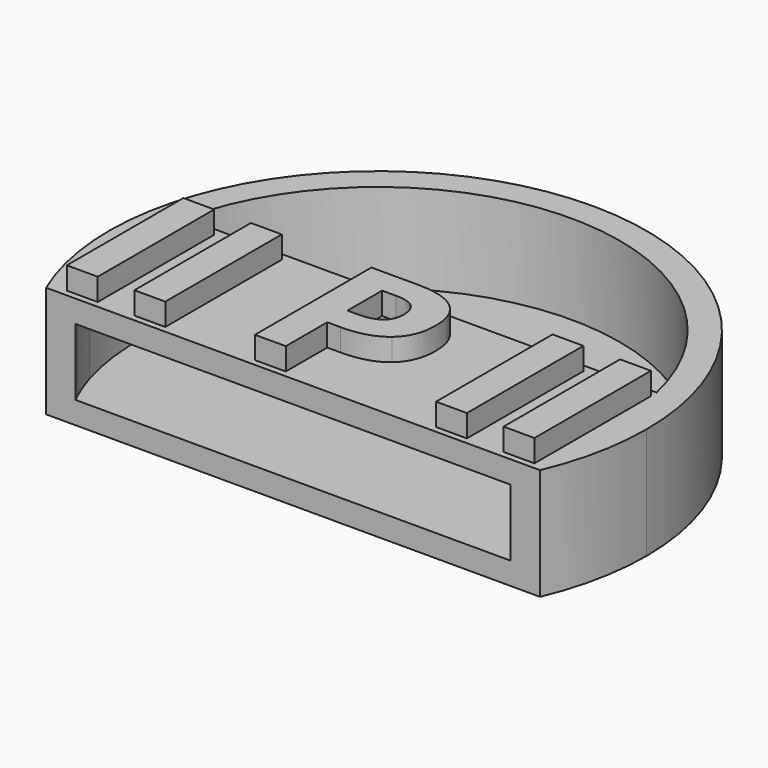
from build123d import *

# Parameters (mm, degrees)
F0_W     = 1.3848739799
F0_H     = 6.5299166297
F1_DEPTH = 5
F2_DEPTH = 6
F3_DEPTH = 4
F4_DEPTH = 1


# Not quite as in the source:
# - a feature names something its author has since deleted; it is built from what else it names


with BuildPart() as f1:
    # F0 (on Top) → F1 (new body)
    with BuildSketch(Plane.XY):
        with BuildLine():
            ThreePointArc((-9.8874952566, -4.4676545918), (-9.8222615585, -4.6093034047), (-9.7549987186, -4.75))
            Line((-9.7549987186, -4.75), (9.7549987186, -4.75))
            ThreePointArc((9.7549987186, -4.75), (9.8222615585, -4.6093034047), (9.8874952566, -4.4676545918))
            Line((9.8874952566, -4.4676545918), (9.2131992894, -4.4676545918))
            Line((9.2131992894, -4.4676545918), (9.2131992894, 2.062262038))
            Line((9.2131992894, 2.062262038), (10.5980732693, 2.062262038))
            Line((10.5980732693, 2.062262038), (10.5980732693, -2.3245091907))
            ThreePointArc((10.5980732693, -2.3245091907), (10.7868344516, -1.1690605262), (10.85, 0))
            ThreePointArc((10.85, 0), (10.7825989969, 1.2075010861), (10.5812333875, 2.4))
            Line((10.5812333875, 2.4), (0, 2.4))
            Line((0, 2.4), (-10.5812333875, 2.4))
            ThreePointArc((-10.5812333875, 2.4), (-10.8422277422, -0.4106063639), (-10.3694047071, -3.1934223053))
            Line((-10.3694047071, -3.1934223053), (-10.3694047071, 2.062262038))
            Line((-10.3694047071, 2.062262038), (-8.9845307272, 2.062262038))
            Line((-8.9845307272, 2.062262038), (-8.9845307272, -4.4676545918))
            Line((-8.9845307272, -4.4676545918), (-9.8874952566, -4.4676545918))
        make_face()
        with Locations((-6.6485384464, -1.2026962769)):
            Rectangle(F0_W, F0_H, mode=Mode.SUBTRACT)
        with BuildLine():
            add(Edge.make_bspline(
                [(1.9565453854, 1.55061613), (2.5746650927, 1.0389702221), (2.5746650927, 0.0256826557)],
                knots=[0, 0, 0, 1, 1, 1], degree=2))
            add(Edge.make_bspline(
                [(2.5746650927, 0.0256826557), (2.5746650927, -1.0290510875), (1.9158137978, -1.5871452971)],
                knots=[0, 0, 0, 1, 1, 1], degree=2))
            add(Edge.make_bspline(
                [(1.9158137978, -1.5871452971), (1.2569625029, -2.1452395068), (0.0421607662, -2.1452395068)],
                knots=[0, 0, 0, 1, 1, 1], degree=2))
            Line((0.0421607662, -2.1452395068), (-0.5509483171, -2.1452395068))
            Line((-0.5509483171, -2.1452395068), (-0.5509483171, -4.4676545918))
            Line((-0.5509483171, -4.4676545918), (-1.935822297, -4.4676545918))
            Line((-1.935822297, -4.4676545918), (-1.935822297, 2.062262038))
            Line((-1.935822297, 2.062262038), (0.1493491547, 2.062262038))
            add(Edge.make_bspline(
                [(0.1493491547, 2.062262038), (1.3384256782, 2.062262038), (1.9565453854, 1.55061613)],
                knots=[0, 0, 0, 1, 1, 1], degree=2))
        make_face(mode=Mode.SUBTRACT)
        with Locations((6.8772070086, -1.2026962769)):
            Rectangle(F0_W, F0_H, mode=Mode.SUBTRACT)
        with BuildLine():
            ThreePointArc((11.0742945599, -4.75), (11.8035534787, -2.4245876508), (12.05, 0))
            ThreePointArc((12.05, 0), (-2.4245876508, 11.8035534787), (-11.0742945599, -4.75))
            Line((-11.0742945599, -4.75), (-9.7549987186, -4.75))
            ThreePointArc((-9.7549987186, -4.75), (-9.8222615585, -4.6093034047), (-9.8874952566, -4.4676545918))
            Line((-9.8874952566, -4.4676545918), (-10.3694047071, -4.4676545918))
            Line((-10.3694047071, -4.4676545918), (-10.3694047071, -3.1934223053))
            ThreePointArc((-10.3694047071, -3.1934223053), (-10.8422277422, -0.4106063639), (-10.5812333875, 2.4))
            ThreePointArc((-10.5812333875, 2.4), (0, 10.85), (10.5812333875, 2.4))
            ThreePointArc((10.5812333875, 2.4), (10.7825989969, 1.2075010861), (10.85, 0))
            ThreePointArc((10.85, 0), (10.7868344516, -1.1690605262), (10.5980732693, -2.3245091907))
            Line((10.5980732693, -2.3245091907), (10.5980732693, -4.4676545918))
            Line((10.5980732693, -4.4676545918), (9.8874952566, -4.4676545918))
            ThreePointArc((9.8874952566, -4.4676545918), (9.8222615585, -4.6093034047), (9.7549987186, -4.75))
            Line((9.7549987186, -4.75), (11.0742945599, -4.75))
        make_face()
        with BuildLine():
            Line((-0.5509483171, 0.927494298), (-0.5509483171, -1.0104717668))
            Line((-0.5509483171, -1.0104717668), (-0.0950403712, -1.0104717668))
            add(Edge.make_bspline(
                [(-0.0950403712, -1.0104717668), (0.542373246, -1.0104717668), (0.8596508761, -0.7582217591)],
                knots=[0, 0, 0, 1, 1, 1], degree=2))
            add(Edge.make_bspline(
                [(0.8596508761, -0.7582217591), (1.1769285061, -0.5059717514), (1.1769285061, -0.0243385922)],
                knots=[0, 0, 0, 1, 1, 1], degree=2))
            add(Edge.make_bspline(
                [(1.1769285061, -0.0243385922), (1.1769285061, 0.463011281), (0.9111013026, 0.6952527895)],
                knots=[0, 0, 0, 1, 1, 1], degree=2))
            add(Edge.make_bspline(
                [(0.9111013026, 0.6952527895), (0.645274099, 0.927494298), (0.077890229, 0.927494298)],
                knots=[0, 0, 0, 1, 1, 1], degree=2))
            Line((0.077890229, 0.927494298), (-0.5509483171, 0.927494298))
        make_face()
    extrude(amount=F1_DEPTH)

    # F0 (on Top) → F2 (join)
    with BuildSketch(Plane.XY):
        with BuildLine():
            ThreePointArc((-10.3694047071, -3.1934223053), (-10.1484686537, -3.8381094285), (-9.8874952566, -4.4676545918))
            Line((-9.8874952566, -4.4676545918), (-8.9845307272, -4.4676545918))
            Line((-8.9845307272, -4.4676545918), (-8.9845307272, 2.062262038))
            Line((-8.9845307272, 2.062262038), (-10.3694047071, 2.062262038))
            Line((-10.3694047071, 2.062262038), (-10.3694047071, -3.1934223053))
        make_face()
        with BuildLine():
            Line((-10.3694047071, -4.4676545918), (-9.8874952566, -4.4676545918))
            ThreePointArc((-9.8874952566, -4.4676545918), (-10.1484686537, -3.8381094285), (-10.3694047071, -3.1934223053))
            Line((-10.3694047071, -3.1934223053), (-10.3694047071, -4.4676545918))
        make_face()
        with Locations((-6.6485384464, -1.2026962769)):
            Rectangle(F0_W, F0_H)
        with BuildLine():
            add(Edge.make_bspline(
                [(2.5746650927, 0.0256826557), (2.5746650927, -1.0290510875), (1.9158137978, -1.5871452971)],
                knots=[0, 0, 0, 1, 1, 1], degree=2))
            add(Edge.make_bspline(
                [(1.9565453854, 1.55061613), (2.5746650927, 1.0389702221), (2.5746650927, 0.0256826557)],
                knots=[0, 0, 0, 1, 1, 1], degree=2))
            add(Edge.make_bspline(
                [(0.1493491547, 2.062262038), (1.3384256782, 2.062262038), (1.9565453854, 1.55061613)],
                knots=[0, 0, 0, 1, 1, 1], degree=2))
            Line((0.1493491547, 2.062262038), (-1.935822297, 2.062262038))
            Line((-1.935822297, 2.062262038), (-1.935822297, -4.4676545918))
            Line((-1.935822297, -4.4676545918), (-0.5509483171, -4.4676545918))
            Line((-0.5509483171, -4.4676545918), (-0.5509483171, -2.1452395068))
            Line((-0.5509483171, -2.1452395068), (0.0421607662, -2.1452395068))
            add(Edge.make_bspline(
                [(1.9158137978, -1.5871452971), (1.2569625029, -2.1452395068), (0.0421607662, -2.1452395068)],
                knots=[0, 0, 0, 1, 1, 1], degree=2))
        make_face()
        with BuildLine():
            Line((-0.0950403712, -1.0104717668), (-0.5509483171, -1.0104717668))
            Line((-0.5509483171, -1.0104717668), (-0.5509483171, 0.927494298))
            Line((-0.5509483171, 0.927494298), (0.077890229, 0.927494298))
            add(Edge.make_bspline(
                [(0.9111013026, 0.6952527895), (0.645274099, 0.927494298), (0.077890229, 0.927494298)],
                knots=[0, 0, 0, 1, 1, 1], degree=2))
            add(Edge.make_bspline(
                [(1.1769285061, -0.0243385922), (1.1769285061, 0.463011281), (0.9111013026, 0.6952527895)],
                knots=[0, 0, 0, 1, 1, 1], degree=2))
            add(Edge.make_bspline(
                [(0.8596508761, -0.7582217591), (1.1769285061, -0.5059717514), (1.1769285061, -0.0243385922)],
                knots=[0, 0, 0, 1, 1, 1], degree=2))
            add(Edge.make_bspline(
                [(-0.0950403712, -1.0104717668), (0.542373246, -1.0104717668), (0.8596508761, -0.7582217591)],
                knots=[0, 0, 0, 1, 1, 1], degree=2))
        make_face(mode=Mode.SUBTRACT)
        with Locations((6.8772070086, -1.2026962769)):
            Rectangle(F0_W, F0_H)
        with BuildLine():
            Line((9.2131992894, -4.4676545918), (9.8874952566, -4.4676545918))
            ThreePointArc((9.8874952566, -4.4676545918), (10.2986842611, -3.4146160092), (10.5980732693, -2.3245091907))
            Line((10.5980732693, -2.3245091907), (10.5980732693, 2.062262038))
            Line((10.5980732693, 2.062262038), (9.2131992894, 2.062262038))
            Line((9.2131992894, 2.062262038), (9.2131992894, -4.4676545918))
        make_face()
        with BuildLine():
            ThreePointArc((10.5980732693, -2.3245091907), (10.2986842611, -3.4146160092), (9.8874952566, -4.4676545918))
            Line((9.8874952566, -4.4676545918), (10.5980732693, -4.4676545918))
            Line((10.5980732693, -4.4676545918), (10.5980732693, -2.3245091907))
        make_face()
    extrude(amount=F2_DEPTH)

    # F0 (on Top) → F3 (cut)
    with BuildSketch(Plane.XY):
        with BuildLine():
            ThreePointArc((-9.8874952566, -4.4676545918), (-9.8222615585, -4.6093034047), (-9.7549987186, -4.75))
            Line((-9.7549987186, -4.75), (9.7549987186, -4.75))
            ThreePointArc((9.7549987186, -4.75), (9.8222615585, -4.6093034047), (9.8874952566, -4.4676545918))
            Line((9.8874952566, -4.4676545918), (9.2131992894, -4.4676545918))
            Line((9.2131992894, -4.4676545918), (9.2131992894, 2.062262038))
            Line((9.2131992894, 2.062262038), (10.5980732693, 2.062262038))
            Line((10.5980732693, 2.062262038), (10.5980732693, -2.3245091907))
            ThreePointArc((10.5980732693, -2.3245091907), (10.7868344516, -1.1690605262), (10.85, 0))
            ThreePointArc((10.85, 0), (10.7825989969, 1.2075010861), (10.5812333875, 2.4))
            Line((10.5812333875, 2.4), (0, 2.4))
            Line((0, 2.4), (-10.5812333875, 2.4))
            ThreePointArc((-10.5812333875, 2.4), (-10.8422277422, -0.4106063639), (-10.3694047071, -3.1934223053))
            Line((-10.3694047071, -3.1934223053), (-10.3694047071, 2.062262038))
            Line((-10.3694047071, 2.062262038), (-8.9845307272, 2.062262038))
            Line((-8.9845307272, 2.062262038), (-8.9845307272, -4.4676545918))
            Line((-8.9845307272, -4.4676545918), (-9.8874952566, -4.4676545918))
        make_face()
        with Locations((-6.6485384464, -1.2026962769)):
            Rectangle(F0_W, F0_H, mode=Mode.SUBTRACT)
        with BuildLine():
            add(Edge.make_bspline(
                [(1.9565453854, 1.55061613), (2.5746650927, 1.0389702221), (2.5746650927, 0.0256826557)],
                knots=[0, 0, 0, 1, 1, 1], degree=2))
            add(Edge.make_bspline(
                [(2.5746650927, 0.0256826557), (2.5746650927, -1.0290510875), (1.9158137978, -1.5871452971)],
                knots=[0, 0, 0, 1, 1, 1], degree=2))
            add(Edge.make_bspline(
                [(1.9158137978, -1.5871452971), (1.2569625029, -2.1452395068), (0.0421607662, -2.1452395068)],
                knots=[0, 0, 0, 1, 1, 1], degree=2))
            Line((0.0421607662, -2.1452395068), (-0.5509483171, -2.1452395068))
            Line((-0.5509483171, -2.1452395068), (-0.5509483171, -4.4676545918))
            Line((-0.5509483171, -4.4676545918), (-1.935822297, -4.4676545918))
            Line((-1.935822297, -4.4676545918), (-1.935822297, 2.062262038))
            Line((-1.935822297, 2.062262038), (0.1493491547, 2.062262038))
            add(Edge.make_bspline(
                [(0.1493491547, 2.062262038), (1.3384256782, 2.062262038), (1.9565453854, 1.55061613)],
                knots=[0, 0, 0, 1, 1, 1], degree=2))
        make_face(mode=Mode.SUBTRACT)
        with Locations((6.8772070086, -1.2026962769)):
            Rectangle(F0_W, F0_H, mode=Mode.SUBTRACT)
        with BuildLine():
            ThreePointArc((-10.3694047071, -3.1934223053), (-10.1484686537, -3.8381094285), (-9.8874952566, -4.4676545918))
            Line((-9.8874952566, -4.4676545918), (-8.9845307272, -4.4676545918))
            Line((-8.9845307272, -4.4676545918), (-8.9845307272, 2.062262038))
            Line((-8.9845307272, 2.062262038), (-10.3694047071, 2.062262038))
            Line((-10.3694047071, 2.062262038), (-10.3694047071, -3.1934223053))
        make_face()
        with Locations((-6.6485384464, -1.2026962769)):
            Rectangle(F0_W, F0_H)
        with BuildLine():
            add(Edge.make_bspline(
                [(2.5746650927, 0.0256826557), (2.5746650927, -1.0290510875), (1.9158137978, -1.5871452971)],
                knots=[0, 0, 0, 1, 1, 1], degree=2))
            add(Edge.make_bspline(
                [(1.9565453854, 1.55061613), (2.5746650927, 1.0389702221), (2.5746650927, 0.0256826557)],
                knots=[0, 0, 0, 1, 1, 1], degree=2))
            add(Edge.make_bspline(
                [(0.1493491547, 2.062262038), (1.3384256782, 2.062262038), (1.9565453854, 1.55061613)],
                knots=[0, 0, 0, 1, 1, 1], degree=2))
            Line((0.1493491547, 2.062262038), (-1.935822297, 2.062262038))
            Line((-1.935822297, 2.062262038), (-1.935822297, -4.4676545918))
            Line((-1.935822297, -4.4676545918), (-0.5509483171, -4.4676545918))
            Line((-0.5509483171, -4.4676545918), (-0.5509483171, -2.1452395068))
            Line((-0.5509483171, -2.1452395068), (0.0421607662, -2.1452395068))
            add(Edge.make_bspline(
                [(1.9158137978, -1.5871452971), (1.2569625029, -2.1452395068), (0.0421607662, -2.1452395068)],
                knots=[0, 0, 0, 1, 1, 1], degree=2))
        make_face()
        with BuildLine():
            Line((-0.0950403712, -1.0104717668), (-0.5509483171, -1.0104717668))
            Line((-0.5509483171, -1.0104717668), (-0.5509483171, 0.927494298))
            Line((-0.5509483171, 0.927494298), (0.077890229, 0.927494298))
            add(Edge.make_bspline(
                [(0.9111013026, 0.6952527895), (0.645274099, 0.927494298), (0.077890229, 0.927494298)],
                knots=[0, 0, 0, 1, 1, 1], degree=2))
            add(Edge.make_bspline(
                [(1.1769285061, -0.0243385922), (1.1769285061, 0.463011281), (0.9111013026, 0.6952527895)],
                knots=[0, 0, 0, 1, 1, 1], degree=2))
            add(Edge.make_bspline(
                [(0.8596508761, -0.7582217591), (1.1769285061, -0.5059717514), (1.1769285061, -0.0243385922)],
                knots=[0, 0, 0, 1, 1, 1], degree=2))
            add(Edge.make_bspline(
                [(-0.0950403712, -1.0104717668), (0.542373246, -1.0104717668), (0.8596508761, -0.7582217591)],
                knots=[0, 0, 0, 1, 1, 1], degree=2))
        make_face(mode=Mode.SUBTRACT)
        with BuildLine():
            Line((-0.5509483171, 0.927494298), (-0.5509483171, -1.0104717668))
            Line((-0.5509483171, -1.0104717668), (-0.0950403712, -1.0104717668))
            add(Edge.make_bspline(
                [(-0.0950403712, -1.0104717668), (0.542373246, -1.0104717668), (0.8596508761, -0.7582217591)],
                knots=[0, 0, 0, 1, 1, 1], degree=2))
            add(Edge.make_bspline(
                [(0.8596508761, -0.7582217591), (1.1769285061, -0.5059717514), (1.1769285061, -0.0243385922)],
                knots=[0, 0, 0, 1, 1, 1], degree=2))
            add(Edge.make_bspline(
                [(1.1769285061, -0.0243385922), (1.1769285061, 0.463011281), (0.9111013026, 0.6952527895)],
                knots=[0, 0, 0, 1, 1, 1], degree=2))
            add(Edge.make_bspline(
                [(0.9111013026, 0.6952527895), (0.645274099, 0.927494298), (0.077890229, 0.927494298)],
                knots=[0, 0, 0, 1, 1, 1], degree=2))
            Line((0.077890229, 0.927494298), (-0.5509483171, 0.927494298))
        make_face()
        with Locations((6.8772070086, -1.2026962769)):
            Rectangle(F0_W, F0_H)
        with BuildLine():
            Line((9.2131992894, -4.4676545918), (9.8874952566, -4.4676545918))
            ThreePointArc((9.8874952566, -4.4676545918), (10.2986842611, -3.4146160092), (10.5980732693, -2.3245091907))
            Line((10.5980732693, -2.3245091907), (10.5980732693, 2.062262038))
            Line((10.5980732693, 2.062262038), (9.2131992894, 2.062262038))
            Line((9.2131992894, 2.062262038), (9.2131992894, -4.4676545918))
        make_face()
    extrude(amount=F3_DEPTH, mode=Mode.SUBTRACT)

    # F0 (on Top) → F4 (join)
    with BuildSketch(Plane.XY):
        with BuildLine():
            ThreePointArc((10.5812333875, 2.4), (0, 10.85), (-10.5812333875, 2.4))
            Line((-10.5812333875, 2.4), (0, 2.4))
            Line((0, 2.4), (10.5812333875, 2.4))
        make_face()
        with BuildLine():
            ThreePointArc((2.35, 4.75), (1.6617009358, 3.0882990642), (0, 2.4))
            ThreePointArc((0, 2.4), (-1.6617009358, 6.4117009358), (2.35, 4.75))
        make_face(mode=Mode.SUBTRACT)
        with BuildLine():
            ThreePointArc((-9.8874952566, -4.4676545918), (-9.8222615585, -4.6093034047), (-9.7549987186, -4.75))
            Line((-9.7549987186, -4.75), (9.7549987186, -4.75))
            ThreePointArc((9.7549987186, -4.75), (9.8222615585, -4.6093034047), (9.8874952566, -4.4676545918))
            Line((9.8874952566, -4.4676545918), (9.2131992894, -4.4676545918))
            Line((9.2131992894, -4.4676545918), (9.2131992894, 2.062262038))
            Line((9.2131992894, 2.062262038), (10.5980732693, 2.062262038))
            Line((10.5980732693, 2.062262038), (10.5980732693, -2.3245091907))
            ThreePointArc((10.5980732693, -2.3245091907), (10.7868344516, -1.1690605262), (10.85, 0))
            ThreePointArc((10.85, 0), (10.7825989969, 1.2075010861), (10.5812333875, 2.4))
            Line((10.5812333875, 2.4), (0, 2.4))
            Line((0, 2.4), (-10.5812333875, 2.4))
            ThreePointArc((-10.5812333875, 2.4), (-10.8422277422, -0.4106063639), (-10.3694047071, -3.1934223053))
            Line((-10.3694047071, -3.1934223053), (-10.3694047071, 2.062262038))
            Line((-10.3694047071, 2.062262038), (-8.9845307272, 2.062262038))
            Line((-8.9845307272, 2.062262038), (-8.9845307272, -4.4676545918))
            Line((-8.9845307272, -4.4676545918), (-9.8874952566, -4.4676545918))
        make_face()
        with Locations((-6.6485384464, -1.2026962769)):
            Rectangle(F0_W, F0_H, mode=Mode.SUBTRACT)
        with BuildLine():
            add(Edge.make_bspline(
                [(1.9565453854, 1.55061613), (2.5746650927, 1.0389702221), (2.5746650927, 0.0256826557)],
                knots=[0, 0, 0, 1, 1, 1], degree=2))
            add(Edge.make_bspline(
                [(2.5746650927, 0.0256826557), (2.5746650927, -1.0290510875), (1.9158137978, -1.5871452971)],
                knots=[0, 0, 0, 1, 1, 1], degree=2))
            add(Edge.make_bspline(
                [(1.9158137978, -1.5871452971), (1.2569625029, -2.1452395068), (0.0421607662, -2.1452395068)],
                knots=[0, 0, 0, 1, 1, 1], degree=2))
            Line((0.0421607662, -2.1452395068), (-0.5509483171, -2.1452395068))
            Line((-0.5509483171, -2.1452395068), (-0.5509483171, -4.4676545918))
            Line((-0.5509483171, -4.4676545918), (-1.935822297, -4.4676545918))
            Line((-1.935822297, -4.4676545918), (-1.935822297, 2.062262038))
            Line((-1.935822297, 2.062262038), (0.1493491547, 2.062262038))
            add(Edge.make_bspline(
                [(0.1493491547, 2.062262038), (1.3384256782, 2.062262038), (1.9565453854, 1.55061613)],
                knots=[0, 0, 0, 1, 1, 1], degree=2))
        make_face(mode=Mode.SUBTRACT)
        with Locations((6.8772070086, -1.2026962769)):
            Rectangle(F0_W, F0_H, mode=Mode.SUBTRACT)
        with BuildLine():
            ThreePointArc((-10.3694047071, -3.1934223053), (-10.1484686537, -3.8381094285), (-9.8874952566, -4.4676545918))
            Line((-9.8874952566, -4.4676545918), (-8.9845307272, -4.4676545918))
            Line((-8.9845307272, -4.4676545918), (-8.9845307272, 2.062262038))
            Line((-8.9845307272, 2.062262038), (-10.3694047071, 2.062262038))
            Line((-10.3694047071, 2.062262038), (-10.3694047071, -3.1934223053))
        make_face()
        with Locations((-6.6485384464, -1.2026962769)):
            Rectangle(F0_W, F0_H)
        with BuildLine():
            add(Edge.make_bspline(
                [(2.5746650927, 0.0256826557), (2.5746650927, -1.0290510875), (1.9158137978, -1.5871452971)],
                knots=[0, 0, 0, 1, 1, 1], degree=2))
            add(Edge.make_bspline(
                [(1.9565453854, 1.55061613), (2.5746650927, 1.0389702221), (2.5746650927, 0.0256826557)],
                knots=[0, 0, 0, 1, 1, 1], degree=2))
            add(Edge.make_bspline(
                [(0.1493491547, 2.062262038), (1.3384256782, 2.062262038), (1.9565453854, 1.55061613)],
                knots=[0, 0, 0, 1, 1, 1], degree=2))
            Line((0.1493491547, 2.062262038), (-1.935822297, 2.062262038))
            Line((-1.935822297, 2.062262038), (-1.935822297, -4.4676545918))
            Line((-1.935822297, -4.4676545918), (-0.5509483171, -4.4676545918))
            Line((-0.5509483171, -4.4676545918), (-0.5509483171, -2.1452395068))
            Line((-0.5509483171, -2.1452395068), (0.0421607662, -2.1452395068))
            add(Edge.make_bspline(
                [(1.9158137978, -1.5871452971), (1.2569625029, -2.1452395068), (0.0421607662, -2.1452395068)],
                knots=[0, 0, 0, 1, 1, 1], degree=2))
        make_face()
        with BuildLine():
            Line((-0.0950403712, -1.0104717668), (-0.5509483171, -1.0104717668))
            Line((-0.5509483171, -1.0104717668), (-0.5509483171, 0.927494298))
            Line((-0.5509483171, 0.927494298), (0.077890229, 0.927494298))
            add(Edge.make_bspline(
                [(0.9111013026, 0.6952527895), (0.645274099, 0.927494298), (0.077890229, 0.927494298)],
                knots=[0, 0, 0, 1, 1, 1], degree=2))
            add(Edge.make_bspline(
                [(1.1769285061, -0.0243385922), (1.1769285061, 0.463011281), (0.9111013026, 0.6952527895)],
                knots=[0, 0, 0, 1, 1, 1], degree=2))
            add(Edge.make_bspline(
                [(0.8596508761, -0.7582217591), (1.1769285061, -0.5059717514), (1.1769285061, -0.0243385922)],
                knots=[0, 0, 0, 1, 1, 1], degree=2))
            add(Edge.make_bspline(
                [(-0.0950403712, -1.0104717668), (0.542373246, -1.0104717668), (0.8596508761, -0.7582217591)],
                knots=[0, 0, 0, 1, 1, 1], degree=2))
        make_face(mode=Mode.SUBTRACT)
        with BuildLine():
            Line((-0.5509483171, 0.927494298), (-0.5509483171, -1.0104717668))
            Line((-0.5509483171, -1.0104717668), (-0.0950403712, -1.0104717668))
            add(Edge.make_bspline(
                [(-0.0950403712, -1.0104717668), (0.542373246, -1.0104717668), (0.8596508761, -0.7582217591)],
                knots=[0, 0, 0, 1, 1, 1], degree=2))
            add(Edge.make_bspline(
                [(0.8596508761, -0.7582217591), (1.1769285061, -0.5059717514), (1.1769285061, -0.0243385922)],
                knots=[0, 0, 0, 1, 1, 1], degree=2))
            add(Edge.make_bspline(
                [(1.1769285061, -0.0243385922), (1.1769285061, 0.463011281), (0.9111013026, 0.6952527895)],
                knots=[0, 0, 0, 1, 1, 1], degree=2))
            add(Edge.make_bspline(
                [(0.9111013026, 0.6952527895), (0.645274099, 0.927494298), (0.077890229, 0.927494298)],
                knots=[0, 0, 0, 1, 1, 1], degree=2))
            Line((0.077890229, 0.927494298), (-0.5509483171, 0.927494298))
        make_face()
        with Locations((6.8772070086, -1.2026962769)):
            Rectangle(F0_W, F0_H)
        with BuildLine():
            Line((9.2131992894, -4.4676545918), (9.8874952566, -4.4676545918))
            ThreePointArc((9.8874952566, -4.4676545918), (10.2986842611, -3.4146160092), (10.5980732693, -2.3245091907))
            Line((10.5980732693, -2.3245091907), (10.5980732693, 2.062262038))
            Line((10.5980732693, 2.062262038), (9.2131992894, 2.062262038))
            Line((9.2131992894, 2.062262038), (9.2131992894, -4.4676545918))
        make_face()
    extrude(amount=F4_DEPTH)


solid = f1.part
